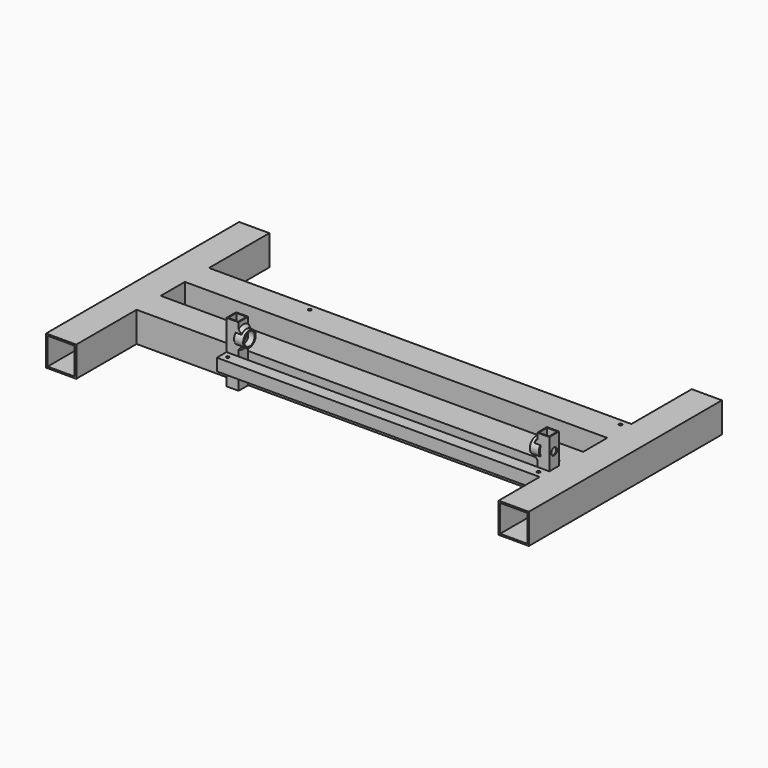
from build123d import *

# Parameters (mm, degrees)
F0_W          = 50
F0_H          = 50
F0_W_2        = 45
F0_H_2        = 45
F1_DEPTH      = 200
F2_W          = 50
F2_H          = 50
F2_W_2        = 45
F2_H_2        = 45
F3_DEPTH      = 700
F4_W          = 20
F4_H          = 20
F4_W_2        = 17
F4_H_2        = 17
F5_DEPTH      = 50
F6_DEPTH      = 50
F7_W          = 20
F7_H          = 20
F7_W_2        = 17
F7_H_2        = 17
F8_DEPTH      = 535
F9_R          = 6
F10_DEPTH     = 750.001
F11_R         = 13
F11_R_2       = 11
F12_DEPTH     = 10
F13_DEPTH     = 5
F14_R         = 13
F14_R_2       = 11
F15_DEPTH     = 10
F16_DEPTH     = 5
F17_T4_ANGLE  = 213.9701071651
F17_T10_ANGLE = 213.9701071651
F17_T16_ANGLE = 213.9701071651
F17_T22_ANGLE = 213.9701071651
F18_R         = 2.5
F19_DEPTH     = 10


# Not quite as in the source:
# - a fillet or chamfer that OpenCascade refuses, or shapes differently, is made with other operations: its cross-section is extruded or revolved along the edge and cut away or added


with BuildPart() as f1:
    # F0 (on Front) → F1 (new body, symmetric)
    with BuildSketch(Plane.XZ):
        with Locations((-375, 0)):
            Rectangle(F0_W, F0_H)
        with Locations((-375, 0)):
            Rectangle(F0_W_2, F0_H_2, mode=Mode.SUBTRACT)
    extrude(amount=F1_DEPTH, both=True)



with BuildPart() as f1b:
    # F0 (on Front) → F1, piece 2 (new body, symmetric)
    with BuildSketch(Plane.XZ):
        with Locations((375, 0)):
            Rectangle(F0_W, F0_H)
        with Locations((375, 0)):
            Rectangle(F0_W_2, F0_H_2, mode=Mode.SUBTRACT)
    extrude(amount=F1_DEPTH, both=True)


with BuildPart() as f1_1:
    add(f1.part)

    add(f1b.part)  # F3 merges F1b
    # F2 (on face) → F3 (join, through all)
    with BuildSketch(Plane.YZ.offset(-350)):
        with Locations((50, 0)):
            Rectangle(F2_W, F2_H)
        with Locations((50, 0)):
            Rectangle(F2_W_2, F2_H_2, mode=Mode.SUBTRACT)
        with Locations((-50, 0)):
            Rectangle(F2_W, F2_H)
        with Locations((-50, 0)):
            Rectangle(F2_W_2, F2_H_2, mode=Mode.SUBTRACT)
    extrude(amount=F3_DEPTH)

    # F4 (on face) → F5 (join)
    with BuildSketch(Plane.XY.offset(25)):
        with Locations((340, -85)):
            Rectangle(F4_W, F4_H)
        with Locations((340, -85)):
            Rectangle(F4_W_2, F4_H_2, mode=Mode.SUBTRACT)
        with Locations((-175, -85)):
            Rectangle(F4_W, F4_H)
        with Locations((-175, -85)):
            Rectangle(F4_W_2, F4_H_2, mode=Mode.SUBTRACT)
    extrude(amount=-F5_DEPTH)

    # F4 (on face) → F6 (join)
    with BuildSketch(Plane.XY.offset(25)):
        with Locations((340, -85)):
            Rectangle(F4_W, F4_H)
        with Locations((340, -85)):
            Rectangle(F4_W_2, F4_H_2, mode=Mode.SUBTRACT)
        with Locations((-175, -85)):
            Rectangle(F4_W, F4_H)
        with Locations((-175, -85)):
            Rectangle(F4_W_2, F4_H_2, mode=Mode.SUBTRACT)
    extrude(amount=F6_DEPTH)

    # F7 (on face) → F8 (join)
    with BuildSketch(Plane(origin=(350, 0, 0), x_dir=(0, -1, 0), z_dir=(-1, 0, 0))):
        with Locations((105, 15)):
            Rectangle(F7_W, F7_H)
        with Locations((105, 15)):
            Rectangle(F7_W_2, F7_H_2, mode=Mode.SUBTRACT)
    extrude(amount=F8_DEPTH)

    # F9 (on face) → F10 (cut, through all)
    with BuildSketch(Plane.YZ.offset(350)):
        with Locations((-85, 50)):
            Circle(F9_R)
    extrude(amount=-F10_DEPTH, mode=Mode.SUBTRACT)

    # F11 (on face) → F12 (join)
    with BuildSketch(Plane(origin=(330, 0, 0), x_dir=(0, -1, 0), z_dir=(-1, 0, 0))):
        with Locations((85, 50)):
            Circle(F11_R)
        with Locations((85, 50)):
            Circle(F11_R_2, mode=Mode.SUBTRACT)
    extrude(amount=F12_DEPTH)

    # F11 (on face) → F13 (join)
    with BuildSketch(Plane(origin=(330, 0, 0), x_dir=(0, -1, 0), z_dir=(-1, 0, 0))):
        with Locations((85, 50)):
            Circle(F11_R)
        with Locations((85, 50)):
            Circle(F11_R_2, mode=Mode.SUBTRACT)
    extrude(amount=-F13_DEPTH)

    # F14 (on face) → F15 (join)
    with BuildSketch(Plane.YZ.offset(-165)):
        with Locations((-85, 50)):
            Circle(F14_R)
        with Locations((-85, 50)):
            Circle(F14_R_2, mode=Mode.SUBTRACT)
    extrude(amount=F15_DEPTH)

    # F14 (on face) → F16 (join)
    with BuildSketch(Plane.YZ.offset(-165)):
        with Locations((-85, 50)):
            Circle(F14_R)
        with Locations((-85, 50)):
            Circle(F14_R_2, mode=Mode.SUBTRACT)
    extrude(amount=-F16_DEPTH)

    # F17: chamfer of 5 on 10 edges, made by hand


with BuildPart() as f17_tool2:
    # F17_s3 → F17_t4 (revolve)
    with BuildSketch(Plane(origin=(0, 6.7154986509, 21.9859176279), x_dir=(1, 0, 0), z_dir=(0, 0.2921222291, 0.9563809927))):
        Polygon((-165, -113.8984958377), (-160, -108.8984958377), (-165, -108.8984958377), align=None)
    revolve(axis=Axis((-165, -85, 50), (1, 0, 0)), revolution_arc=F17_T4_ANGLE)

    split(bisect_by=Plane.XZ.offset(75), keep=Keep.TOP)

    split(bisect_by=Plane.XZ.offset(95), keep=Keep.BOTTOM)


with BuildPart() as f1_2:
    add(f1_1.part)

    # F17_t1: union F17_tool2
    add(f17_tool2.part)


with BuildPart() as f17_tool8:
    # F17_s9 → F17_t10 (revolve)
    with BuildSketch(Plane(origin=(0, 6.7154986509, 21.9859176279), x_dir=(1, 0, 0), z_dir=(0, -0.2921222291, -0.9563809927))):
        Polygon((-165, 77.8984958377), (-160, 82.8984958377), (-165, 82.8984958377), align=None)
    revolve(axis=Axis((-165, -85, 50), (1, 0, 0)), revolution_arc=F17_T10_ANGLE)

    split(bisect_by=Plane.XZ.offset(75), keep=Keep.TOP)

    split(bisect_by=Plane.XZ.offset(95), keep=Keep.BOTTOM)


with BuildPart() as f1_3:
    add(f1_2.part)

    # F17_t7: union F17_tool8
    add(f17_tool8.part)


with BuildPart() as f17_tool14:
    # F17_s15 → F17_t16 (revolve)
    with BuildSketch(Plane(origin=(0, -21.2225160964, 69.4805426982), x_dir=(1, 0, 0), z_dir=(0, -0.2921222291, 0.9563809927))):
        Polygon((330, -48.686272927), (325, -53.686272927), (330, -53.686272927), align=None)
    revolve(axis=Axis((330, -85, 50), (-1, 0, 0)), revolution_arc=F17_T16_ANGLE)

    split(bisect_by=Plane.XZ.offset(75), keep=Keep.TOP)

    split(bisect_by=Plane.XZ.offset(95), keep=Keep.BOTTOM)


with BuildPart() as f1_4:
    add(f1_3.part)

    # F17_t13: union F17_tool14
    add(f17_tool14.part)


with BuildPart() as f17_tool20:
    # F17_s21 → F17_t22 (revolve)
    with BuildSketch(Plane(origin=(0, -21.2225160964, 69.4805426982), x_dir=(1, 0, 0), z_dir=(0, 0.2921222291, -0.9563809927))):
        Polygon((330, 84.686272927), (325, 79.686272927), (330, 79.686272927), align=None)
    revolve(axis=Axis((330, -85, 50), (-1, 0, 0)), revolution_arc=F17_T22_ANGLE)

    split(bisect_by=Plane.XZ.offset(75), keep=Keep.TOP)

    split(bisect_by=Plane.XZ.offset(95), keep=Keep.BOTTOM)


with BuildPart() as f1_5:
    add(f1_4.part)

    # F17_t19: union F17_tool20
    add(f17_tool20.part)

    # F18 (on face) → F19 (cut)
    with BuildSketch(Plane.XY.offset(25)):
        with Locations((-175, -65)):
            Circle(F18_R)
        with Locations((-175, 65)):
            Circle(F18_R)
        with Locations((-175, -105)):
            Circle(F18_R)
        with Locations((340, -105)):
            Circle(F18_R)
        with Locations((340, -65)):
            Circle(F18_R)
        with Locations((340, 65)):
            Circle(F18_R)
    extrude(amount=-F19_DEPTH, mode=Mode.SUBTRACT)


solid = f1_5.part
